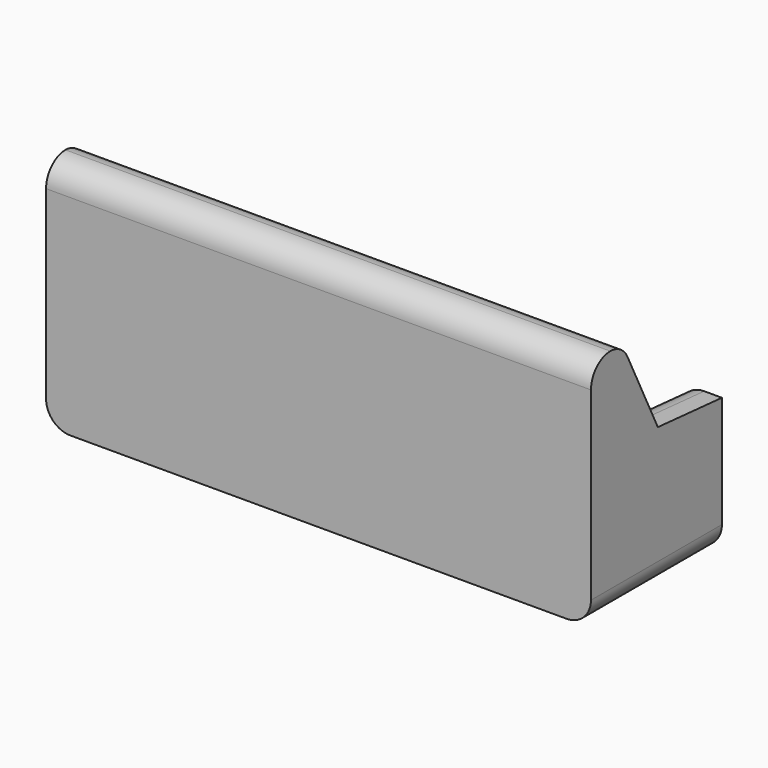
from build123d import *

# Parameters (mm, degrees)
F0_W         = 111.8826307356
F0_H         = 33.61280635
F1_DEPTH     = 48
F3_DEPTH     = 92
F5_DEPTH     = 9
F6_T1_DEPTH  = 94.5960432291
F7_R         = 5
F8_R         = 5
F9_R         = 5
F10_T1_DEPTH = 136.8826307356
F10_T3_DEPTH = 127.4671918099


# Not quite as in the source:
# - a fillet or chamfer that OpenCascade refuses, or shapes differently, is made with other operations: its cross-section is extruded or revolved along the edge and cut away or added


with BuildPart() as f1:
    # F0 (on Top) → F1 (new body)
    with BuildSketch(Plane.XY):
        with Locations((-7.0826988667, -28.0907023698)):
            Rectangle(F0_W, F0_H)
    extrude(amount=F1_DEPTH)

    # F2 (on Right) → F3 (cut, symmetric)
    with BuildSketch(Plane.YZ):
        Polygon((-2.2725867394, 56.280748791), (-39.9752296507, 54.2606711388), (-27.7305655181, 29.2911604047), (-4.6817823313, 27.3704268038), align=None)
    extrude(amount=F3_DEPTH, both=True, mode=Mode.SUBTRACT)

    # F4 (on face) → F5 (cut)
    with BuildSketch(Plane(origin=(0, 2.2328525009, 26.7942067339), x_dir=(1, 0, 0), z_dir=(0, 0.0830455515, 0.9965457523))):
        Polygon((40.2153246105, -5.8544473723), (-54.3807186186, -8.7455315515), (-54.3807186186, -30.0672778452), (40.2153246105, -30.0672778452), align=None)
    extrude(amount=-F5_DEPTH, mode=Mode.SUBTRACT)

    # F6: fillet of radius 53.3943165321 on 1 edges, made by hand

    # F6_s2 → F6_t1 (cut)
    with BuildSketch(Plane.YZ.offset(-54.3807186186)):
        with BuildLine():
            ThreePointArc((-33.8957137688, 41.863227205), (-30.0543394398, 31.3775725516), (-28.4779754817, 20.3222486342))
            Line((-28.4779754817, 20.3222486342), (-27.7305655181, 29.2911604047))
            Line((-27.7305655181, 29.2911604047), (-33.8957137688, 41.863227205))
        make_face()
    extrude(amount=F6_T1_DEPTH, mode=Mode.SUBTRACT)

    # F7
    f7_edges = [f1.edges().sort_by_distance(p)[0] for p in [
        (-54.380719, -19.507432, 28.605899),
        (40.215325, -19.507432, 28.605899),
    ]]
    fillet(f7_edges, radius=F7_R)

    # F8
    f8_edges = [f1.edges().sort_by_distance(p)[0] for p in [
        (-7.082697, -11.284299, 18.889441),
    ]]
    fillet(f8_edges, radius=F8_R)

    # F9
    f9_edges = [f1.edges().sort_by_distance(p)[0] for p in [
        (-63.024014, -28.090702, 0),
        (48.858617, -28.090702, 0),
    ]]
    fillet(f9_edges, radius=F9_R)

    # F10: fillet of radius 5 on 2 edges, made by hand

    # F10_s2 → F10_t1 (cut)
    with BuildSketch(Plane.YZ.offset(-75.5240142345)):
        with BuildLine():
            ThreePointArc((-44.8971055448, 43), (-43.4326394507, 46.5355339059), (-39.8971055448, 48))
            Line((-39.8971055448, 48), (-44.8971055448, 48))
            Line((-44.8971055448, 48), (-44.8971055448, 43))
        make_face()
    extrude(amount=F10_T1_DEPTH, mode=Mode.SUBTRACT)

    # F10_s4 → F10_t3 (cut)
    with BuildSketch(Plane.YZ.offset(-70.8162947717)):
        with BuildLine():
            ThreePointArc((-35.5327359736, 45.2014685051), (-37.3769475866, 47.2430733275), (-40.0220050033, 48))
            Line((-40.0220050033, 48), (-36.9050927884, 48))
            Line((-36.9050927884, 48), (-35.5327359736, 45.2014685051))
        make_face()
    extrude(amount=F10_T3_DEPTH, mode=Mode.SUBTRACT)


solid = f1.part
